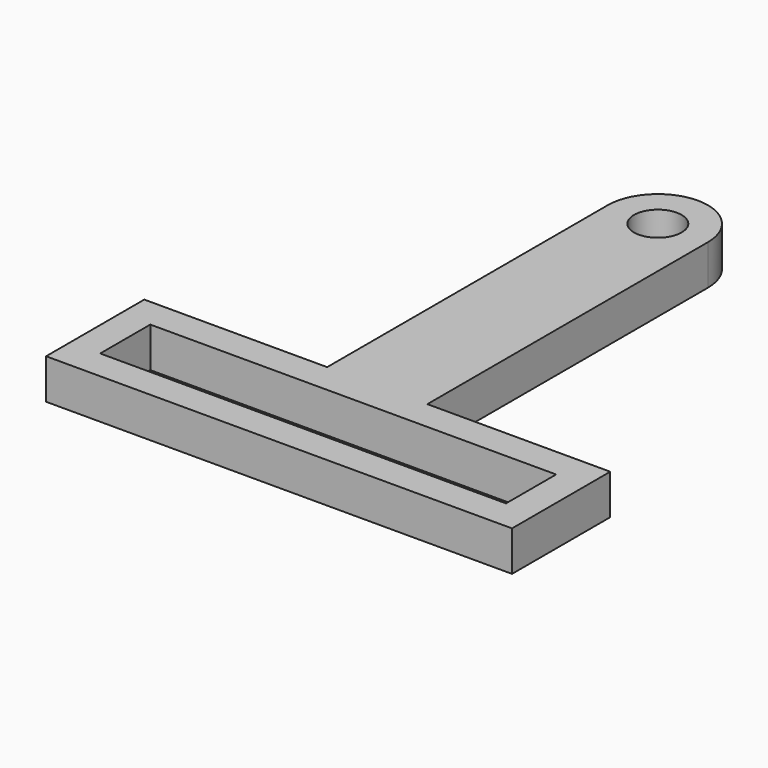
from build123d import *

# Parameters (mm, degrees)
F0_W     = 3
F0_H     = 3
F0_W_2   = 40.5
F0_H_2   = 6.25
F0_W_3   = 10
F0_H_3   = 40
F1_DEPTH = 4
F2_R     = 4.99999
F3_R     = 2.375
F4_DEPTH = 4.001


# Not quite as in the source:
# - a fillet or chamfer is up to 0.001 mm smaller than in the source, because OpenCascade refuses the exact size


with BuildPart() as f1:
    # F0 (on Top) → F1 (new body)
    with BuildSketch(Plane.XY):
        with Locations((21.75, -1.5)):
            Rectangle(F0_W, F0_H)
        Polygon((20.25, -3), (20.25, 0), (5, 0), (-5, 0), (-23.25, 0), (-23.25, -12.25), (23.25, -12.25), (23.25, -3), align=None)
        with Locations((0, -6.125)):
            Rectangle(F0_W_2, F0_H_2, mode=Mode.SUBTRACT)
        with Locations((0, 20)):
            Rectangle(F0_W_3, F0_H_3)
    extrude(amount=F1_DEPTH)

    # F2 (radius 5 in the source; OpenCascade refuses exactly that, so slightly less here)
    f2_edges = [f1.edges().sort_by_distance(p)[0] for p in [
        (5, 40, 2),
        (-5, 40, 2),
    ]]
    fillet(f2_edges, radius=F2_R)

    # F3 (on face) → F4 (cut, through all)
    with BuildSketch(Plane.XY.offset(4)):
        with Locations((0, 35)):
            Circle(F3_R)
    extrude(amount=-F4_DEPTH, mode=Mode.SUBTRACT)


solid = f1.part
